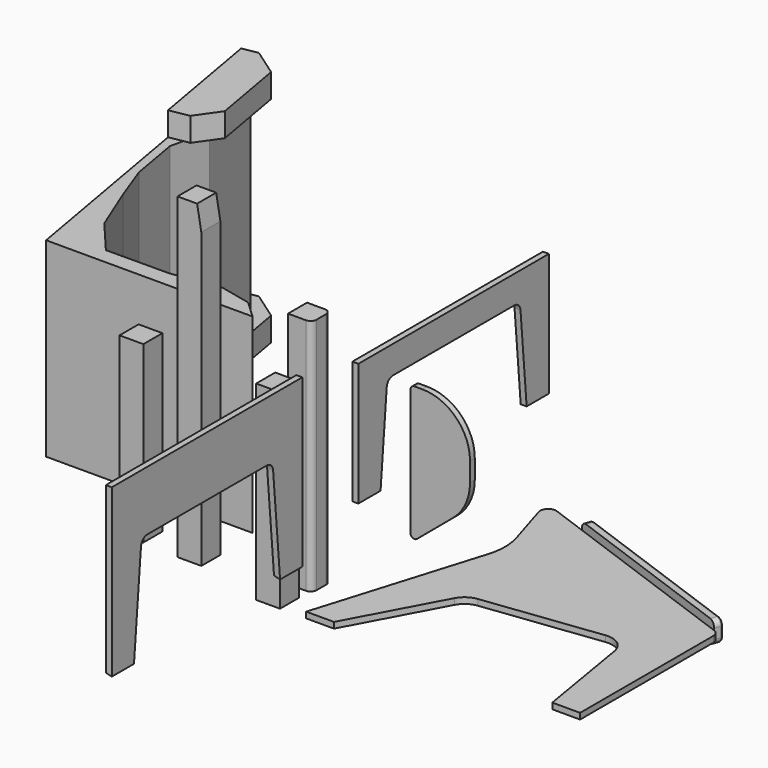
from build123d import *

# Parameters (mm, degrees)
F1_DEPTH    = 15
F3_DEPTH    = 20
F4_R        = 5
F6_DEPTH    = 600
F7_R        = 50
F9_DEPTH    = 300
F10_R       = 10
F12_DEPTH   = 15
F13_SIZE2   = 4.019228
F13_SIZE    = 14.99999
F13_2_SIZE2 = 4.019228
F13_2_SIZE  = 14.99999
F15_W       = 60
F15_H       = 60
F16_DEPTH   = 440
F17_W       = 60
F17_H       = 60
F18_DEPTH   = 800
F19_SIZE2   = 10.5796188425
F19_SIZE    = 60
F20_W       = 60
F20_H       = 60
F21_DEPTH   = 600
F23_DEPTH   = 15
F24_R       = 15
F25_W       = 60
F25_H       = 60
F26_DEPTH   = 480
F28_DEPTH   = 480
F29_W       = 300
F29_H       = 60
F30_DEPTH   = 100
F31_SIZE    = 50
F32_SIZE    = 60


# Not quite as in the source:
# - a fillet or chamfer is up to 0.001 mm smaller than in the source, because OpenCascade refuses the exact size


with BuildPart() as f1:
    # F0 (on Top) → F1 (new body)
    with BuildSketch(Plane.XY):
        with BuildLine():
            Line((126.6180717201, 416.2354741443), (0, 0))
            Line((0, 0), (70, 0))
            Line((70, 0), (191.8851607508, 227.1694949665))
            ThreePointArc((191.8851607508, 227.1694949665), (207.7011825649, 244.7896539907), (229.8505687934, 253.1575234781))
            Line((229.8505687934, 253.1575234781), (523.1229672837, 289.1668461516))
            ThreePointArc((523.1229672837, 289.1668461516), (559.1324176201, 279.6024135438), (578.5306128266, 247.7925266))
            Line((578.5306128266, 247.7925266), (620, 0))
            Line((620, 0), (690, 0))
            Line((690, 0), (690, 420))
            ThreePointArc((690, 420), (686.3830408858, 431.471528727), (676.8404028665, 438.7938524157))
            Line((676.8404028665, 438.7938524157), (117.6946363687, 642.3062680369))
            ThreePointArc((117.6946363687, 642.3062680369), (97.0871419884, 638.0199030414), (91.728138383, 617.6649815267))
            Line((91.728138383, 617.6649815267), (126.5567223416, 503.7458164876))
            ThreePointArc((126.5567223416, 503.7458164876), (133.1109720865, 459.9952186871), (126.6180717201, 416.2354741443))
        make_face()
    extrude(amount=F1_DEPTH)

    # F2 (on face) → F3 (join)
    with BuildSketch(Plane(origin=(220.2009124558, 604.9970347157, 0), x_dir=(-0.9396926208, 0.3420201433, 0), z_dir=(0.3420201433, 0.9396926208, 0))):
        with BuildLine():
            Line((-0.9455957298, 35), (-470.9455957298, 35))
            ThreePointArc((-470.9455957298, 35), (-481.5521974476, 30.6066017178), (-485.9455957298, 20))
            Line((-485.9455957298, 20), (-485.9455957298, -5))
            ThreePointArc((-485.9455957298, -5), (-481.5521974476, -15.6066017178), (-470.9455957298, -20))
            Line((-470.9455957298, -20), (-0.9455957298, -20))
            ThreePointArc((-0.9455957298, -20), (9.661005988, -15.6066017178), (14.0544042702, -5))
            Line((14.0544042702, -5), (14.0544042702, 20))
            ThreePointArc((14.0544042702, 20), (9.661005988, 30.6066017178), (-0.9455957298, 35))
        make_face()
    extrude(amount=F3_DEPTH)

    # F4
    f4_edges = [f1.edges().sort_by_distance(p)[0] for p in [
        (448.757651, 543.092741, -20),
    ]]
    fillet(f4_edges, radius=F4_R)


with BuildPart() as f6:
    # F5 (on Front) → F6 (new body)
    with BuildSketch(Plane.XZ):
        with BuildLine():
            Line((-123.4288864959, -313.8082504272), (0, -1013.8082504272))
            Line((0, -1013.8082504272), (626.6764420045, -1013.8082504272))
            ThreePointArc((626.6764420045, -1013.8082504272), (645.8275530824, -1004.8779406694), (651.2966358298, -984.4670459856))
            Line((651.2966358298, -984.4670459856), (640.3123613054, -922.1721295738))
            ThreePointArc((640.3123613054, -922.1721295738), (604.7540774342, -861.8146206111), (538.3170815047, -839.5987251324))
            Line((538.3170815047, -839.5987251324), (134.2559409884, -853.8082504272))
            Line((134.2559409884, -853.8082504272), (39.0393714058, -313.8082504272))
            Line((39.0393714058, -313.8082504272), (39.0393714058, -13.8082504272))
            Line((39.0393714058, -13.8082504272), (-123.4288864959, -13.8082504272))
            Line((-123.4288864959, -13.8082504272), (-123.4288864959, -313.8082504272))
        make_face()
    extrude(amount=F6_DEPTH)

    # F7
    f7_edges = [f6.edges().sort_by_distance(p)[0] for p in [
        (0, -300, -1013.80825),
    ]]
    fillet(f7_edges, radius=F7_R)

    # F8 (on face) → F9 (join)
    with BuildSketch(Plane.XY.offset(-13.8082504272)):
        Polygon((-123.4288864959, 0), (39.0393714058, 0), (175.9928613901, 89.3815875053), (66.5727051852, 89.3815875053), align=None)
        Polygon((175.9928613901, -689.3815875053), (39.0393714058, -600), (-123.4288864959, -600), (66.5727051852, -689.3815875053), align=None)
    extrude(amount=-F9_DEPTH)

    # F10 (call 1 of 8: OpenCascade refuses the feature's edges together)
    f10_edges = [f6.edges().sort_by_distance(p)[0] for p in [
        (175.992861, -689.381588, -163.80825),
    ]]
    fillet(f10_edges, radius=F10_R)

    # F10#2 (call 2 of 8)
    f10_2_edges = [f6.edges().sort_by_distance(p)[0] for p in [
        (175.992861, 89.381588, -163.80825),
    ]]
    fillet(f10_2_edges, radius=F10_R)

    # F10#3 (call 3 of 8)
    f10_3_edges = [f6.edges().sort_by_distance(p)[0] for p in [
        (66.572705, -689.381588, -163.80825),
    ]]
    fillet(f10_3_edges, radius=F10_R)

    # F10#4 (call 4 of 8)
    f10_4_edges = [f6.edges().sort_by_distance(p)[0] for p in [
        (-123.428886, -600, -163.80825),
    ]]
    fillet(f10_4_edges, radius=F10_R)

    # F10#5 (call 5 of 8)
    f10_5_edges = [f6.edges().sort_by_distance(p)[0] for p in [
        (66.572705, 89.381588, -163.80825),
    ]]
    fillet(f10_5_edges, radius=F10_R)

    # F10#6 (call 6 of 8)
    f10_6_edges = [f6.edges().sort_by_distance(p)[0] for p in [
        (-123.428886, 0, -163.80825),
    ]]
    fillet(f10_6_edges, radius=F10_R)

    # F10#7 (call 7 of 8)
    f10_7_edges = [f6.edges().sort_by_distance(p)[0] for p in [
        (39.039371, -600, -163.80825),
    ]]
    fillet(f10_7_edges, radius=F10_R)

    # F10#8 (call 8 of 8)
    f10_8_edges = [f6.edges().sort_by_distance(p)[0] for p in [
        (39.039371, 0, -163.80825),
    ]]
    fillet(f10_8_edges, radius=F10_R)


with BuildPart() as f12:
    # F11 (on Right) → F12 (new body)
    with BuildSketch(Plane.YZ):
        with BuildLine():
            Line((-30.8854154888, 552.1247227984), (-630.8854154888, 552.1247227984))
            Line((-630.8854154888, 552.1247227984), (-630.8854154888, 132.1247227984))
            Line((-630.8854154888, 132.1247227984), (-560.8854154888, 132.1247227984))
            Line((-560.8854154888, 132.1247227984), (-538.8607468183, 383.8678376533))
            ThreePointArc((-538.8607468183, 383.8678376533), (-532.4486570087, 396.8702695346), (-518.9368528564, 402.1247227984))
            Line((-518.9368528564, 402.1247227984), (-142.8339781211, 402.1247227984))
            ThreePointArc((-142.8339781211, 402.1247227984), (-129.3221739688, 396.8702695346), (-122.9100841593, 383.8678376533))
            Line((-122.9100841593, 383.8678376533), (-100.8854154888, 132.1247227984))
            Line((-100.8854154888, 132.1247227984), (-30.8854154888, 132.1247227984))
            Line((-30.8854154888, 132.1247227984), (-30.8854154888, 552.1247227984))
        make_face()
    extrude(amount=F12_DEPTH)

    # F13 (size 15 and 4.0192378865 in the source; OpenCascade refuses exactly that, so slightly less here)
    f13_edges = [f12.edges().sort_by_distance(p)[0] for p in [
        (0, -595.885415, 132.124723),
    ]]
    f13_side = f12.faces().sort_by_distance((7.5, -595.885415, 132.124723))[0]
    chamfer(f13_edges, length=F13_SIZE, length2=F13_SIZE2, reference=f13_side)

    # F13#2 (size 15 and 4.0192378865 in the source; OpenCascade refuses exactly that, so slightly less here)
    f13_2_edges = [f12.edges().sort_by_distance(p)[0] for p in [
        (0, -65.885415, 132.124723),
    ]]
    f13_2_side = f12.faces().sort_by_distance((7.5, -65.885415, 132.124723))[0]
    chamfer(f13_2_edges, length=F13_2_SIZE, length2=F13_2_SIZE2, reference=f13_2_side)


with BuildPart() as f12b:
    # F11 (on Right) → F12, piece 2 (new body)
    with BuildSketch(Plane.YZ):
        with BuildLine():
            Line((745.5232589184, 510.3265881046), (145.5232589184, 510.3265881046))
            Line((145.5232589184, 510.3265881046), (145.5232589184, 200.3265881046))
            Line((145.5232589184, 200.3265881046), (215.5232589184, 200.3265881046))
            Line((215.5232589184, 200.3265881046), (234.9232676831, 422.0697029596))
            ThreePointArc((234.9232676831, 422.0697029596), (241.3353574927, 435.0721348408), (254.847161645, 440.3265881046))
            Line((254.847161645, 440.3265881046), (636.1993561918, 440.3265881046))
            ThreePointArc((636.1993561918, 440.3265881046), (649.7111603441, 435.0721348408), (656.1232501537, 422.0697029596))
            Line((656.1232501537, 422.0697029596), (675.5232589184, 200.3265881046))
            Line((675.5232589184, 200.3265881046), (745.5232589184, 200.3265881046))
            Line((745.5232589184, 200.3265881046), (745.5232589184, 510.3265881046))
        make_face()
    extrude(amount=F12_DEPTH)


with BuildPart() as f16:
    # F15 (on Top) → F16 (new body)
    with BuildSketch(Plane.XY):
        with Locations((-481.9470045646, 82.3008220813)):
            Rectangle(F15_W, F15_H)
    extrude(amount=F16_DEPTH)


with BuildPart() as f18:
    # F17 (on Top) → F18 (new body)
    with BuildSketch(Plane.XY):
        with Locations((-330.7043761015, 75.7473593429)):
            Rectangle(F17_W, F17_H)
    extrude(amount=F18_DEPTH)

    # F19
    f19_edges = [f18.edges().sort_by_distance(p)[0] for p in [
        (-300.704376, 75.747359, 800),
    ]]
    f19_side = f18.faces().sort_by_distance((-300.704376, 75.747359, 400))[0]
    chamfer(f19_edges, length=F19_SIZE, length2=F19_SIZE2, reference=f19_side)


with BuildPart() as f21:
    # F20 (on Top) → F21 (new body)
    with BuildSketch(Plane.XY):
        with Locations((-89.059138, 121.5652438998)):
            Rectangle(F20_W, F20_H)
    extrude(amount=F21_DEPTH)

    # F24
    f24_edges = [f21.edges().sort_by_distance(p)[0] for p in [
        (-59.059138, 151.565244, 300),
        (-59.059138, 91.565244, 300),
    ]]
    fillet(f24_edges, radius=F24_R)


with BuildPart() as f23:
    # F22 (on Front) → F23 (new body)
    with BuildSketch(Plane.XZ):
        with BuildLine():
            Line((304.7723621194, 613.257972736), (284.7723621194, 613.257972736))
            ThreePointArc((284.7723621194, 613.257972736), (277.7012943075, 610.3290405479), (274.7723621194, 603.257972736))
            Line((274.7723621194, 603.257972736), (274.7723621194, 284.7030419411))
            ThreePointArc((274.7723621194, 284.7030419411), (280.546179502, 275.6399640708), (291.2002382162, 277.0425975099))
            Line((291.2002382162, 277.0425975099), (381.9068752817, 353.154503217))
            ThreePointArc((381.9068752817, 353.154503217), (413.5292965638, 394.3656449823), (424.7723621194, 445.0798363912))
            Line((424.7723621194, 445.0798363912), (424.7723621194, 493.257972736))
            ThreePointArc((424.7723621194, 493.257972736), (389.6251758617, 578.1107864784), (304.7723621194, 613.257972736))
        make_face()
    extrude(amount=F23_DEPTH)


with BuildPart() as f26:
    # F25 (on Top) → F26 (new body)
    with BuildSketch(Plane.XY):
        with Locations((-95.9075767291, 30)):
            Rectangle(F25_W, F25_H)
    extrude(amount=F26_DEPTH)


with BuildPart() as f28:
    # F27 (on Top) → F28 (new body)
    with BuildSketch(Plane.XY):
        Polygon((-829.8647016287, 218.3535151119), (-309.8647016287, 218.3535151119), (-353.7943065166, 259.6203386784), (-431.4419031143, 277.1183550358), (-553.3201474993, 259.6203386784), (-711.8040919304, 259.0134441853), (-785.6842875481, 346.5096950531), (-833.3225846291, 464.4245803356), (-868.1723905917, 558.7047001621), (-890.2310729027, 683.8057041168), (-868.1723905917, 780.8460277596), (-904.6863913536, 956.2211632729), (-968.7832437622, 1006.1997175217), align=None)
    extrude(amount=F28_DEPTH)

    # F29 (on face) → F30 (join)
    with BuildSketch(Plane(origin=(-767.5005687328, -135.3310579767, 0), x_dir=(0.1736481777, -0.984807753, 0), z_dir=(-0.984807753, -0.1736481777, 0))):
        with Locations((-1009.1407277276, -30)):
            Rectangle(F29_W, F29_H)
        with Locations((-1009.1407277276, 510)):
            Rectangle(F29_W, F29_H)
    extrude(amount=-F30_DEPTH)

    # F31
    f31_edges = [f28.edges().sort_by_distance(p)[0] for p in [
        (-818.208015, 728.122209, 510),
        (-818.208015, 728.122209, -30),
    ]]
    chamfer(f31_edges, length=F31_SIZE)

    # F32
    f32_edges = [f28.edges().sort_by_distance(p)[0] for p in [
        (-870.302468, 1023.564535, 510),
        (-870.302468, 1023.564535, -30),
    ]]
    chamfer(f32_edges, length=F32_SIZE)


solid = Compound([f1.part, f12.part, f12b.part, f16.part, f18.part, f21.part, f23.part, f26.part, f28.part])
